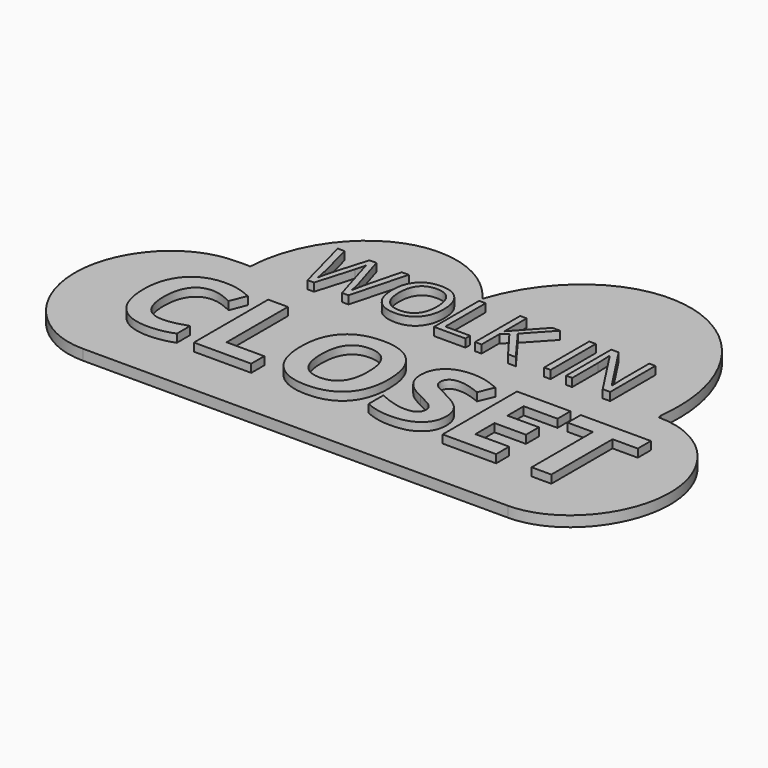
from build123d import *

# Parameters (mm, degrees)
F1_DEPTH       = 2.6
F2_TEXT_SIZE   = 19.5285681593
F2_TEXT_SIZE_2 = 32.1473419841
F3_DEPTH       = 2


# Not quite as in the source:
# - Text() gives the source's letters only with a copy of the font that has no kerning and outlines rounded to 1/6400 em; it was checked with that copy


with BuildPart() as f1:
    # F0 (on Top) → F1 (new body)
    with BuildSketch(Plane.XY):
        with BuildLine():
            Line((-52.479812, -43.617312), (52.479813, -43.617312))
            add(Edge.make_bspline(
                [(73.536525, -19.778938), (73.536525, -32.21635), (64.141991, -43.617312), (52.479813, -43.617312)],
                knots=[0, 0, 0, 0, 1, 1, 1, 1], degree=3))
            add(Edge.make_bspline(
                [(52.317837, 3.368466), (63.980018, 3.368466), (73.536525, -7.514269), (73.536525, -19.778938)],
                knots=[0, 0, 0, 0, 1, 1, 1, 1], degree=3))
            add(Edge.make_bspline(
                [(51.993888, 4.059433), (52.155861, 4.059433), (52.155861, 3.368466), (52.317837, 3.368466)],
                knots=[0, 0, 0, 0, 1, 1, 1, 1], degree=3))
            add(Edge.make_bspline(
                [(52.317837, 9.241688), (52.317837, 7.514268), (52.155861, 5.614108), (51.993888, 4.059433)],
                knots=[0, 0, 0, 0, 1, 1, 1, 1], degree=3))
            add(Edge.make_bspline(
                [(22.676463, 43.617311), (39.035909, 43.617311), (52.317837, 28.243287), (52.317837, 9.241688)],
                knots=[0, 0, 0, 0, 1, 1, 1, 1], degree=3))
            add(Edge.make_bspline(
                [(-5.345164, 20.81539), (-1.133822, 33.943769), (9.880459, 43.617311), (22.676463, 43.617311)],
                knots=[0, 0, 0, 0, 1, 1, 1, 1], degree=3))
            add(Edge.make_bspline(
                [(-24.134233, 30.834414), (-16.521421, 30.834414), (-9.880458, 27.034094), (-5.345164, 20.81539)],
                knots=[0, 0, 0, 0, 1, 1, 1, 1], degree=3))
            add(Edge.make_bspline(
                [(-48.754391, 3.368466), (-48.106493, 18.569745), (-37.254185, 30.834414), (-24.134233, 30.834414)],
                knots=[0, 0, 0, 0, 1, 1, 1, 1], degree=3))
            add(Edge.make_bspline(
                [(-52.479812, 3.368466), (-51.184014, 3.368466), (-50.050189, 3.541208), (-48.754391, 3.368466)],
                knots=[0, 0, 0, 0, 1, 1, 1, 1], degree=3))
            add(Edge.make_bspline(
                [(-73.536525, -19.778938), (-73.536525, -7.341529), (-64.14199, 3.368466), (-52.479812, 3.368466)],
                knots=[0, 0, 0, 0, 1, 1, 1, 1], degree=3))
            add(Edge.make_bspline(
                [(-52.479812, -43.617312), (-64.144784, -43.617312), (-73.536525, -32.21635), (-73.536525, -19.778938)],
                knots=[0, 0, 0, 0, 1, 1, 1, 1], degree=3))
        make_face()
    extrude(amount=F1_DEPTH)

    # F2 (on face) → F3 (join)
    with BuildSketch(Plane.XY.offset(2.6)):
        with Locations((-38.1075815153, 2.8265456106)):
            Text('WOLK IN', F2_TEXT_SIZE, font='Open Sans', text_align=(TextAlign.LEFT, TextAlign.BOTTOM))
        with Locations((-58.3672299981, -31.2146320939)):
            Text('CLOSET', F2_TEXT_SIZE_2, font='Open Sans', font_style=FontStyle.BOLD, text_align=(TextAlign.LEFT, TextAlign.BOTTOM))
    extrude(amount=F3_DEPTH)


solid = f1.part
